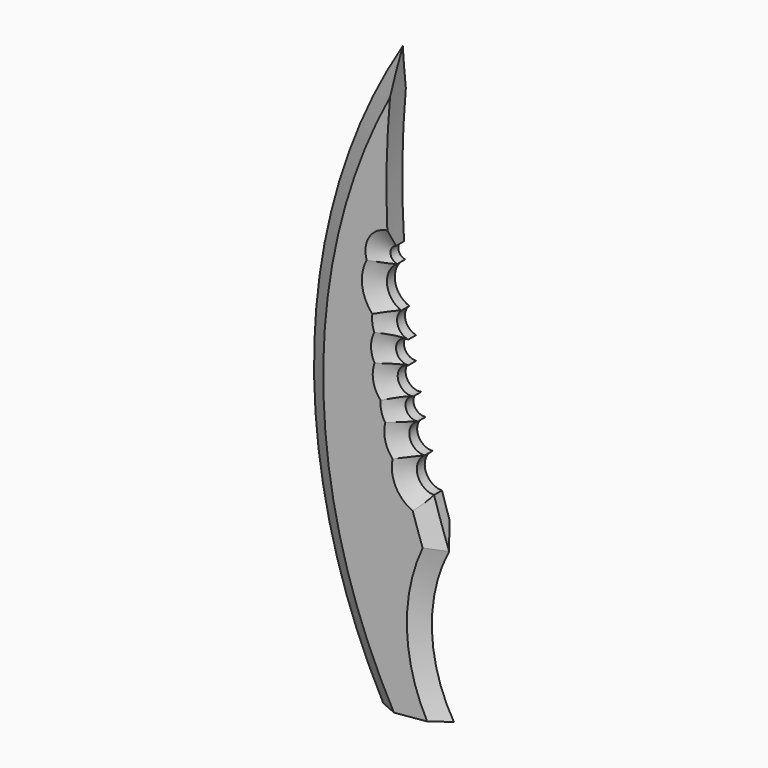
from build123d import *

# Parameters (mm, degrees)
F1_DEPTH    = 1.27
F2_T2_ANGLE = 70.6982594797
F2_T4_ANGLE = 98.1015766654
F2_T6_ANGLE = 98.1015766654
F2_T8_ANGLE = 70.6982594797
F3_SIZE2    = 1.26999
F3_SIZE     = 2.199695


# Not quite as in the source:
# - a fillet or chamfer that OpenCascade refuses, or shapes differently, is made with other operations: its cross-section is extruded or revolved along the edge and cut away or added
# - a fillet or chamfer is up to 0.001 mm smaller than in the source, because OpenCascade refuses the exact size


with BuildPart() as f1:
    # F0 (on Front) → F1 (new body, symmetric)
    with BuildSketch(Plane.XZ):
        with BuildLine():
            ThreePointArc((-24.6599751414, 18.9685343092), (-24.7897166458, 30.8482925644), (-23.6891379404, 42.6776719046))
            ThreePointArc((-23.6891379404, 42.6776719046), (-35.4977812157, 5.0650277845), (-26.6841664691, -33.3599022584))
            Line((-26.6841664691, -33.3599022584), (-16.8598182499, -32.4707999825))
            ThreePointArc((-16.8598182499, -32.4707999825), (-19.7060260634, -23.2610213965), (-17.6819246262, -13.836376369))
            ThreePointArc((-17.6819246262, -13.836376369), (-18.7784432725, -10.7577001108), (-19.7867489636, -7.6490154569))
            ThreePointArc((-19.7867489636, -7.6490154569), (-21.9116415788, -6.0429526618), (-20.9683603212, -3.5520036866))
            ThreePointArc((-20.9683603212, -3.5520036866), (-22.9156863653, -2.1532182096), (-21.8610153861, 0))
            ThreePointArc((-21.8610153861, 0), (-23.4214756824, 1.0408615122), (-22.4479204638, 2.6441765967))
            ThreePointArc((-22.4479204638, 2.6441765967), (-24.4256582154, 3.9784606628), (-23.0913741493, 5.9561984144))
            ThreePointArc((-23.0913741493, 5.9561984144), (-24.6734313076, 7.4086637933), (-23.0913741493, 8.8611291721))
            ThreePointArc((-23.0913741493, 8.8611291721), (-24.4648932463, 10.085402282), (-23.9908037994, 11.8632207636))
            ThreePointArc((-23.9908037994, 11.8632207636), (-25.8325317785, 14.2467515683), (-24.515682055, 16.9558266598))
            ThreePointArc((-24.515682055, 16.9558266598), (-25.3917786695, 17.9045444751), (-24.6599751414, 18.9685343092))
        make_face()
    extrude(amount=F1_DEPTH, both=True)

    # F2: chamfer of 2.54 x 1.4664696837 on 4 edges, made by hand

    # F2_s1 → F2_t2 (revolve, cut)
    with BuildSketch(Plane(origin=(15.8164222993, 0, 20.5345022431), x_dir=(0, 1, 0), z_dir=(0.6102111975, 0, 0.7922387862))):
        Polygon((0.1964696837, 45.0964764528), (-1.27, 42.5564764528), (-1.27, 45.0964764528), align=None)
    revolve(axis=Axis((39.7484673267, -1.27, 2.1011686196), (0, -1, 0)), revolution_arc=F2_T2_ANGLE, mode=Mode.SUBTRACT)

    # F2_s3 → F2_t4 (revolve, cut)
    with BuildSketch(Plane(origin=(10.5087646573, 0, -8.3360437766), x_dir=(0, 1, 0), z_dir=(0.7834430035, 0, -0.6214636436))):
        Polygon((0.1964696837, -37.0387129854), (-1.27, -39.5787129854), (-1.27, -37.0387129854), align=None)
    revolve(axis=Axis((-0.664029112, -1.27, -22.4209338555), (0, 1, 0)), revolution_arc=F2_T4_ANGLE, mode=Mode.SUBTRACT)

    # F2_s5 → F2_t6 (revolve, cut)
    with BuildSketch(Plane(origin=(10.5087646573, 0, -8.3360437766), x_dir=(0, 1, 0), z_dir=(0.7834430035, 0, -0.6214636436))):
        Polygon((-0.1964696837, -37.0387129854), (1.27, -39.5787129854), (1.27, -37.0387129854), align=None)
    revolve(axis=Axis((-0.664029112, 1.27, -22.4209338555), (0, 1, 0)), revolution_arc=F2_T6_ANGLE, mode=Mode.SUBTRACT)

    # F2_s7 → F2_t8 (revolve, cut)
    with BuildSketch(Plane(origin=(15.8164222993, 0, 20.5345022431), x_dir=(0, 1, 0), z_dir=(0.6102111975, 0, 0.7922387862))):
        Polygon((-0.1964696837, 45.0964764528), (1.27, 42.5564764528), (1.27, 45.0964764528), align=None)
    revolve(axis=Axis((39.7484673267, 1.27, 2.1011686196), (0, -1, 0)), revolution_arc=F2_T8_ANGLE, mode=Mode.SUBTRACT)

    # F3 (size 2.1997045256 and 1.27 in the source; OpenCascade refuses exactly that, so slightly less here)
    f3_edges = [f1.edges().sort_by_distance(p)[0] for p in [
        (-25.391779, -1.27, 17.904544),
        (-25.832532, -1.27, 14.246752),
        (-24.464893, -1.27, 10.085402),
        (-24.673431, -1.27, 7.408664),
        (-24.425658, -1.27, 3.978461),
        (-23.421476, -1.27, 1.040862),
        (-22.915686, -1.27, -2.153218),
        (-21.911642, -1.27, -6.042953),
        (-19.304708, -1.27, -9.17292),
    ]]
    f3_side = f1.faces().sort_by_distance((-26.820245, -1.27, -2.285194))[0]
    chamfer(f3_edges, length=F3_SIZE, length2=F3_SIZE2, reference=f3_side)


solid = f1.part
